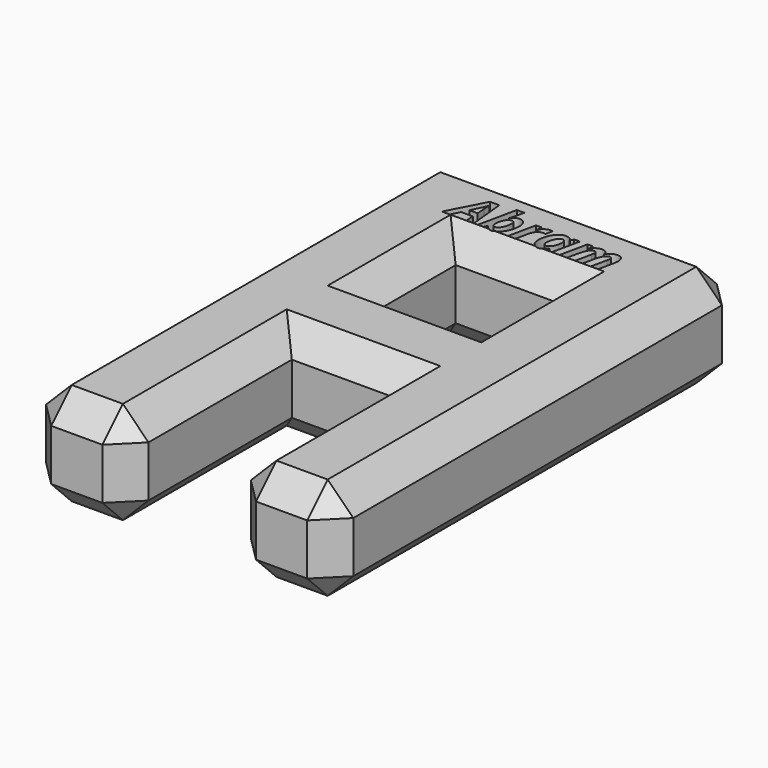
from build123d import *

# Parameters (mm, degrees)
F0_W         = 15.24
F0_H         = 25.4
F1_DEPTH     = 5.08
F2_W         = 5.08
F2_H         = 5.08
F2_H_2       = 10.16
F3_DEPTH     = 5.08
F4_SIZE      = 1.27
F5_TEXT_SIZE = 2.5181826523
F6_DEPTH     = 1.27


# Not quite as in the source:
# - Text() gives the source's letters only with a copy of the font that has no kerning and outlines rounded to 1/6400 em; it was checked with that copy


with BuildPart() as f1:
    # F0 (on Top) → F1 (new body)
    with BuildSketch(Plane.XY):
        Rectangle(F0_W, F0_H)
    extrude(amount=F1_DEPTH)

    # F2 (on face) → F3 (cut)
    with BuildSketch(Plane.XY.offset(5.08)):
        with Locations((0, 5.08)):
            Rectangle(F2_W, F2_H)
        with Locations((0, -7.62)):
            Rectangle(F2_W, F2_H_2)
    extrude(amount=-F3_DEPTH, mode=Mode.SUBTRACT)

    # F4
    f4_edges = [f1.edges().sort_by_distance(p)[0] for p in [
        (-2.54, 5.08, 5.08),
        (0, 7.62, 5.08),
        (2.54, 5.08, 5.08),
        (0, 2.54, 5.08),
        (0, -2.54, 5.08),
        (-2.54, -7.62, 5.08),
        (5.08, -12.7, 5.08),
        (2.54, -7.62, 5.08),
        (-5.08, -12.7, 5.08),
        (-7.62, 0, 5.08),
        (0, 12.7, 5.08),
        (7.62, 0, 5.08),
        (-2.54, -12.7, 2.54),
        (-7.62, -12.7, 2.54),
        (2.54, -12.7, 2.54),
        (7.62, -12.7, 2.54),
        (7.62, 12.7, 2.54),
        (-7.62, 12.7, 2.54),
        (0, 12.7, 0),
        (-2.54, 5.08, 0),
        (2.54, 5.08, 0),
        (0, 7.62, 0),
        (0, 2.54, 0),
        (0, -2.54, 0),
        (-2.54, -7.62, 0),
        (2.54, -7.62, 0),
        (-7.62, 0, 0),
        (7.62, 0, 0),
        (-5.08, -12.7, 0),
        (5.08, -12.7, 0),
    ]]
    chamfer(f4_edges, length=F4_SIZE)

    # F5 (on face) → F6 (cut)
    with BuildSketch(Plane.XY.offset(5.08)):
        with Locations((-4.0857230779, 8.89)):
            Text('Abram', F5_TEXT_SIZE, font='Open Sans', font_style=FontStyle.BOLDITALIC, text_align=(TextAlign.LEFT, TextAlign.BOTTOM))
    extrude(amount=-F6_DEPTH, mode=Mode.SUBTRACT)


solid = f1.part
